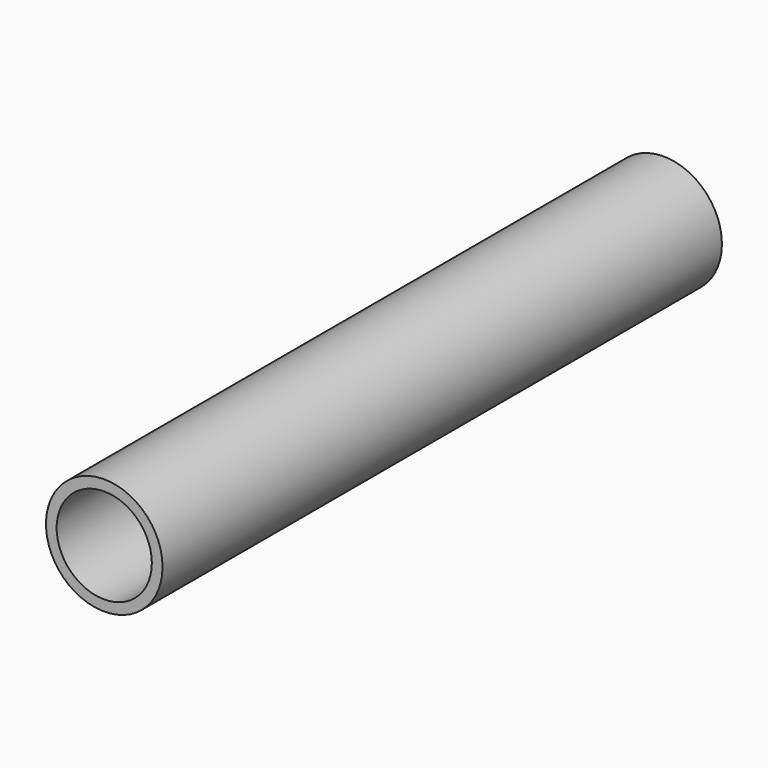
from build123d import *

# Parameters (mm, degrees)
F0_R     = 15
F1_DEPTH = 180
F2_R     = 12.25
F3_DEPTH = 180
F4_R     = 12.25
F5_DEPTH = 180


# Not quite as in the source:
# - the program builds the solid bodies; features that only make, move or delete a surface that nothing else refers to are left out


with BuildPart() as f1:
    # F0 (on Front) → F1 (new body)
    with BuildSketch(Plane.XZ):
        Circle(F0_R)
    extrude(amount=F1_DEPTH)

    # F2 (on Front) → F3 (cut)
    with BuildSketch(Plane.XZ):
        Circle(F2_R)
    extrude(amount=-F3_DEPTH, mode=Mode.SUBTRACT)

    # F4 (on Front) → F5 (cut)
    with BuildSketch(Plane.XZ):
        Circle(F4_R)
    extrude(amount=F5_DEPTH, mode=Mode.SUBTRACT)


solid = f1.part
